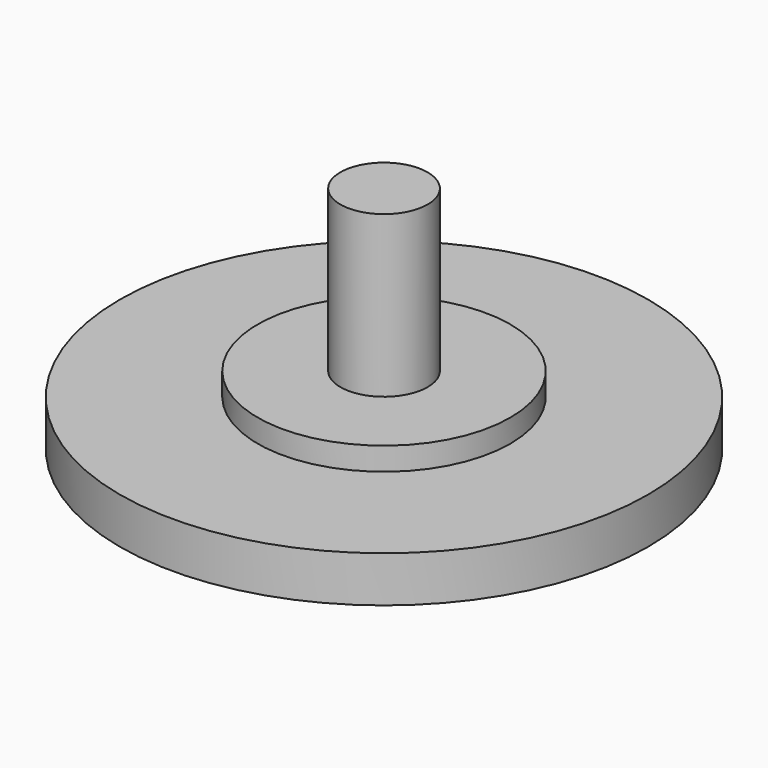
from build123d import *

# Parameters (mm, degrees)
F0_R         = 11.5
F1_DEPTH     = 2
F2_R         = 5.5
F3_DEPTH     = 1
F4_R         = 1.9
F5_DEPTH     = 7
F6_TEXT_SIZE = 17.1190625729
F7_DEPTH     = 1


# Not quite as in the source:
# - Text() gives the source's letters only with a copy of the font that has no kerning and outlines rounded to 1/6400 em; it was checked with that copy


with BuildPart() as f1:
    # F0 (on Top) → F1 (new body)
    with BuildSketch(Plane.XY):
        Circle(F0_R)
    extrude(amount=F1_DEPTH)

    # F2 (on face) → F3 (join)
    with BuildSketch(Plane.XY.offset(2)):
        Circle(F2_R)
    extrude(amount=F3_DEPTH)

    # F4 (on face) → F5 (join)
    with BuildSketch(Plane.XY.offset(3)):
        Circle(F4_R)
    extrude(amount=F5_DEPTH)

    # F6 (on face) → F7 (cut)
    with BuildSketch(Plane(origin=(0, 0, 0), x_dir=(1, 0, 0), z_dir=(0, 0, -1))):
        with Locations((-5.201873706, -6.5597926368)):
            Text('P', F6_TEXT_SIZE, font='Open Sans', text_align=(TextAlign.LEFT, TextAlign.BOTTOM))
    extrude(amount=-F7_DEPTH, mode=Mode.SUBTRACT)


solid = f1.part
